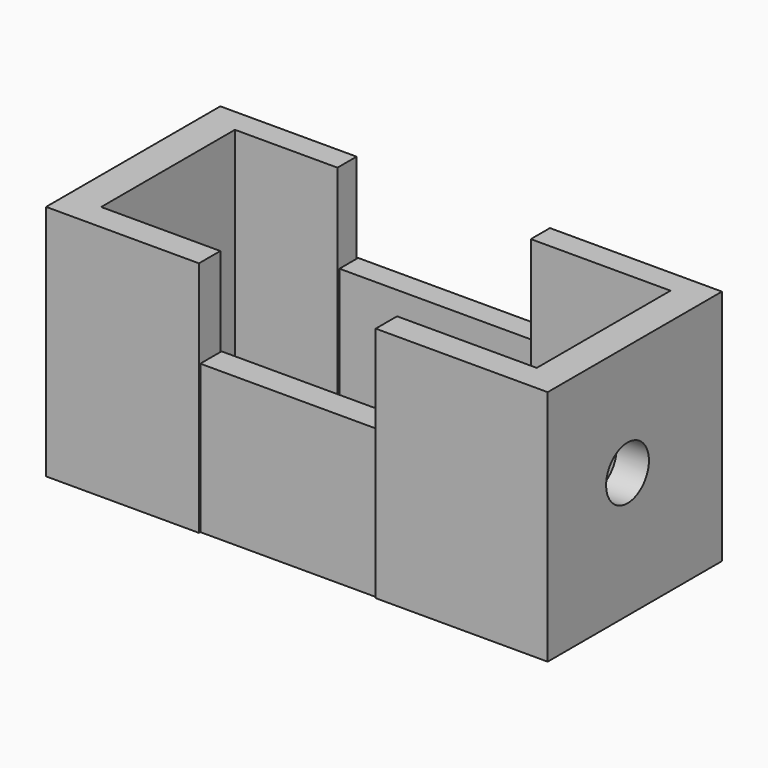
from build123d import *

# Parameters (mm, degrees)
F1_DEPTH = 50.8
F2_W     = 41.4717281237
F2_H     = 4.9982732162
F3_DEPTH = 31.75
F2_W_2   = 38.1761500612
F2_H_2   = 5.6986734271
F4_R     = 5.7287532934
F5_DEPTH = 127
F6_R     = 5.4312735945
F7_DEPTH = 25.4


with BuildPart() as f1:
    # F0 (on Top) → F1 (new body)
    with BuildSketch(Plane.XY):
        Polygon((-23.6167833209, 19.4009207189), (-52.7885518968, 19.4009207189), (-52.7885518968, -27.2214487195), (-20.0658570975, -27.2214487195), (-20.0658570975, -21.506447345), (-45.5696061254, -21.506447345), (-45.5696061254, 14.2875006422), (-23.6167833209, 14.2875006422), align=None)
    extrude(amount=F1_DEPTH)

    # F6 (on face) → F7 (cut)
    with BuildSketch(Plane(origin=(-52.7885518968, 0, 0), x_dir=(0, -1, 0), z_dir=(-1, 0, 0))):
        with Locations((3.9102640003, 25.3669396043)):
            Circle(F6_R)
    extrude(amount=-F7_DEPTH, mode=Mode.SUBTRACT)


with BuildPart() as f1b:
    # F0 (on Top) → F1, piece 2 (new body)
    with BuildSketch(Plane.XY):
        Polygon((54.5932911336, 19.4009207189), (17.7750429139, 19.4009207189), (17.7750429139, 14.2875006422), (47.6751327515, 14.2875006422), (47.6751327515, -21.506447345), (17.7750429139, -21.506447345), (17.7750429139, -27.2214487195), (54.5932911336, -27.2214487195), align=None)
    extrude(amount=F1_DEPTH)

    # F4 (on face) → F5 (cut)
    with BuildSketch(Plane.YZ.offset(54.5932911336)):
        with Locations((-5.8620786294, 26.9034262747)):
            Circle(F4_R)
    extrude(amount=-F5_DEPTH, mode=Mode.SUBTRACT)


with BuildPart() as f3:
    # F2 (on Top) → F3 (new body)
    with BuildSketch(Plane.XY):
        with Locations((-2.6350240223, 17.0118384995)):
            Rectangle(F2_W, F2_H)
    extrude(amount=F3_DEPTH)


with BuildPart() as f3b:
    # F2 (on Top) → F3, piece 2 (new body)
    with BuildSketch(Plane.XY):
        with Locations((-0.987234991, -24.0153409541)):
            Rectangle(F2_W_2, F2_H_2)
    extrude(amount=F3_DEPTH)


solid = Compound([f1.part, f1b.part, f3.part, f3b.part])
